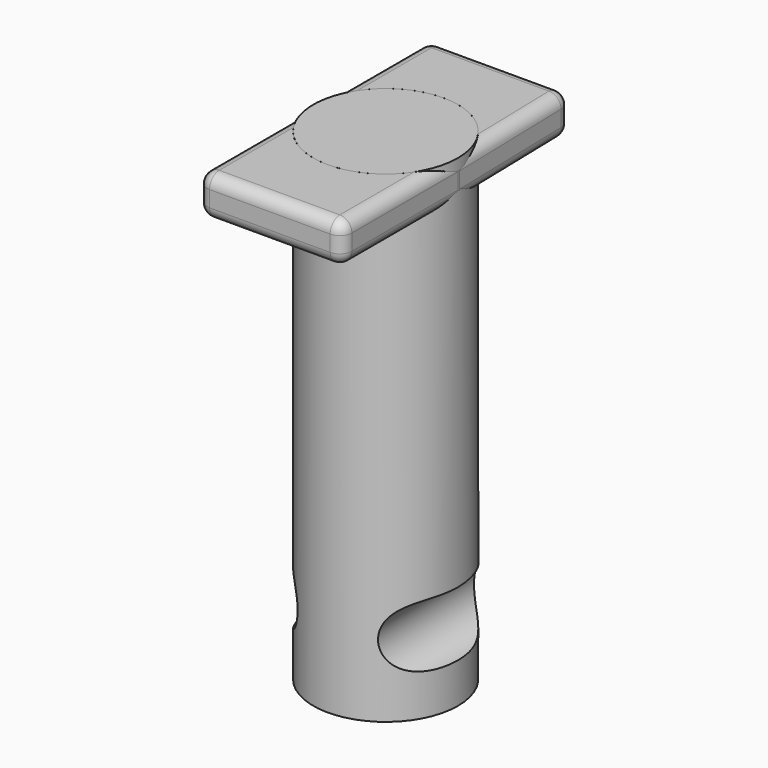
from build123d import *

# Parameters (mm, degrees)
F0_R          = 9
F1_DEPTH      = 60
F2_R          = 4
F3_DEPTH      = 12.55118
F3_DEPTH_BACK = 46.0374
F5_DEPTH      = 5
F6_T1_DEPTH   = 22.875
F6_T3_DEPTH   = 20.25
F6_T5_DEPTH   = 15.002743
F6_T7_DEPTH   = 2
F6_S11_W      = 1.5
F6_S11_H      = 1.5
F6_T12_DEPTH  = 1.5
F6_S17_W      = 1.5
F6_S17_H      = 1.5
F6_T18_DEPTH  = 1.5
F6_S23_W      = 1.5
F6_S23_H      = 1.5
F6_T24_DEPTH  = 1.5
F6_S29_W      = 1.5
F6_S29_H      = 1.5
F6_T30_DEPTH  = 1.5
F6_2_F1_R     = 1.5
F6_2_F2_R     = 1.5
F6_2_F3_R     = 1.5
F6_2_F4_R     = 1.5


# Not quite as in the source:
# - a fillet or chamfer that OpenCascade refuses, or shapes differently, is made with other operations: its cross-section is extruded or revolved along the edge and cut away or added


with BuildPart() as f1:
    # F0 (on Top) → F1 (new body)
    with BuildSketch(Plane.XY):
        Circle(F0_R)
    extrude(amount=F1_DEPTH)

    # F2 (on Front) → F3 (cut, two sides)
    with BuildSketch(Plane.XZ) as f3_sk:
        with Locations((-8.93038, 9)):
            Circle(F2_R)
        with Locations((9.026195, 9)):
            Circle(F2_R)
    extrude(amount=F3_DEPTH, mode=Mode.SUBTRACT)
    extrude(f3_sk.sketch, amount=-F3_DEPTH_BACK, mode=Mode.SUBTRACT)


with BuildPart() as f5:
    # F4 (on face) → F5 (new body)
    with BuildSketch(Plane.XY.offset(60)):
        with BuildLine():
            ThreePointArc((9, 0), (0, -9), (-9, 0))
            Line((-9, 0), (-9, -18))
            Line((-9, -18), (9.002743, -18))
            Line((9.002743, -18), (9.002743, 0))
            Line((9.002743, 0), (8.997257, 0.222169))
            ThreePointArc((8.997257, 0.222169), (8.999314, 0.111093), (9, 0))
        make_face()
    extrude(amount=-F5_DEPTH)

    # F6: fillet of radius 1.5 on 8 edges, made by hand

    # F6_s2 → F6_t1 (cut)
    with BuildSketch(Plane.XZ.offset(-6.375)):
        with BuildLine():
            ThreePointArc((-7.5, 60), (-8.56066, 59.56066), (-9, 58.5))
            Line((-9, 58.5), (-9, 60))
            Line((-9, 60), (-7.5, 60))
        make_face()
        with BuildLine():
            ThreePointArc((-9, 56.5), (-8.56066, 55.43934), (-7.5, 55))
            Line((-7.5, 55), (-9, 55))
            Line((-9, 55), (-9, 56.5))
        make_face()
    extrude(amount=F6_T1_DEPTH, mode=Mode.SUBTRACT)

    # F6_s4 → F6_t3 (cut)
    with BuildSketch(Plane.XZ.offset(-3.75)):
        with BuildLine():
            ThreePointArc((7.502743, 60), (8.563404, 59.56066), (9.002743, 58.5))
            Line((9.002743, 58.5), (9.002743, 60))
            Line((9.002743, 60), (7.502743, 60))
        make_face()
        with BuildLine():
            ThreePointArc((9.002743, 56.5), (8.563404, 55.43934), (7.502743, 55))
            Line((7.502743, 55), (9.002743, 55))
            Line((9.002743, 55), (9.002743, 56.5))
        make_face()
    extrude(amount=F6_T3_DEPTH, mode=Mode.SUBTRACT)

    # F6_s6 → F6_t5 (cut)
    with BuildSketch(Plane.YZ.offset(-7.5)):
        with BuildLine():
            ThreePointArc((-16.5, 60), (-17.56066, 59.56066), (-18, 58.5))
            Line((-18, 58.5), (-18, 60))
            Line((-18, 60), (-16.5, 60))
        make_face()
        with BuildLine():
            ThreePointArc((-18, 56.5), (-17.56066, 55.43934), (-16.5, 55))
            Line((-16.5, 55), (-18, 55))
            Line((-18, 55), (-18, 56.5))
        make_face()
    extrude(amount=F6_T5_DEPTH, mode=Mode.SUBTRACT)

    # F6_s8 → F6_t7 (cut)
    with BuildSketch(Plane.XY.offset(56.5)):
        with BuildLine():
            ThreePointArc((9.002743, -16.5), (8.563404, -17.56066), (7.502743, -18))
            Line((7.502743, -18), (9.002743, -18))
            Line((9.002743, -18), (9.002743, -16.5))
        make_face()
        with BuildLine():
            ThreePointArc((-7.5, -18), (-8.56066, -17.56066), (-9, -16.5))
            Line((-9, -16.5), (-9, -18))
            Line((-9, -18), (-7.5, -18))
        make_face()
    extrude(amount=F6_T7_DEPTH, mode=Mode.SUBTRACT)


with BuildPart() as f5b:
    # F4 (on face) → F5, piece 2 (new body)
    with BuildSketch(Plane.XY.offset(60)):
        with BuildLine():
            Line((-9, 18), (-9, 0))
            ThreePointArc((-9, 0), (-0.111093, 8.999314), (8.997257, 0.222169))
            Line((8.997257, 0.222169), (8.558269, 18))
            Line((8.558269, 18), (-9, 18))
        make_face()
    extrude(amount=-F5_DEPTH)

    # F6#2: fillet of radius 1.5 on 8 edges, made by hand

    # F6_2_f1
    f6_2_f1_edges = [f5b.edges().sort_by_distance(p)[0] for p in [
        (8.558269, 18, 57.5),
    ]]
    fillet(f6_2_f1_edges, radius=F6_2_F1_R)

    # F6_2_f2
    f6_2_f2_edges = [f5b.edges().sort_by_distance(p)[0] for p in [
        (8.795826, 8.379599, 60),
    ]]
    fillet(f6_2_f2_edges, radius=F6_2_F2_R)

    # F6_2_f3
    f6_2_f3_edges = [f5b.edges().sort_by_distance(p)[0] for p in [
        (8.795826, 8.379599, 55),
    ]]
    fillet(f6_2_f3_edges, radius=F6_2_F3_R)

    # F6_2_f4
    f6_2_f4_edges = [f5b.edges().sort_by_distance(p)[0] for p in [
        (-9, 18, 57.5),
    ]]
    fillet(f6_2_f4_edges, radius=F6_2_F4_R)


with BuildPart() as f6_tool10:
    # F6_s11 → F6_t12 (new body)
    with BuildSketch(Plane.XY.offset(58.5)):
        with Locations((-8.25, -17.25)):
            Rectangle(F6_S11_W, F6_S11_H)
    extrude(amount=F6_T12_DEPTH)

    # F6_s13 → F6_t14 (revolve, cut)
    with BuildSketch(Plane(origin=(-7.5, -16.5, 58.5), x_dir=(0.707107, 0.707107, 0), z_dir=(0.707107, -0.707107, 0))):
        with BuildLine():
            ThreePointArc((0, -1.5), (1.5, 0), (0, 1.5))
            Line((0, 1.5), (0, -1.5))
        make_face()
    revolve(axis=Axis((-7.5, -16.5, 58.5), (0, 0, 1)), mode=Mode.SUBTRACT)


with BuildPart() as f5_1:
    add(f5.part)

    # F6_t9: cut F6_tool10
    add(f6_tool10.part, mode=Mode.SUBTRACT)


with BuildPart() as f6_tool16:
    # F6_s17 → F6_t18 (new body)
    with BuildSketch(Plane.XY.offset(58.5)):
        with Locations((8.252743, -17.25)):
            Rectangle(F6_S17_W, F6_S17_H)
    extrude(amount=F6_T18_DEPTH)

    # F6_s19 → F6_t20 (revolve, cut)
    with BuildSketch(Plane(origin=(7.502743, -16.5, 58.5), x_dir=(-0.707107, 0.707107, 0), z_dir=(0.707107, 0.707107, 0))):
        with BuildLine():
            ThreePointArc((0, -1.5), (1.5, 0), (0, 1.5))
            Line((0, 1.5), (0, -1.5))
        make_face()
    revolve(axis=Axis((7.502743, -16.5, 58.5), (0, 0, 1)), mode=Mode.SUBTRACT)


with BuildPart() as f5_2:
    add(f5_1.part)

    # F6_t15: cut F6_tool16
    add(f6_tool16.part, mode=Mode.SUBTRACT)


with BuildPart() as f6_tool22:
    # F6_s23 → F6_t24 (new body)
    with BuildSketch(Plane.XZ.offset(16.5)):
        with Locations((-8.25, 55.75)):
            Rectangle(F6_S23_W, F6_S23_H)
    extrude(amount=F6_T24_DEPTH)

    # F6_s25 → F6_t26 (revolve, cut)
    with BuildSketch(Plane(origin=(-7.5, -16.5, 56.5), x_dir=(0.707107, 0, 0.707107), z_dir=(0.707107, 0, -0.707107))):
        with BuildLine():
            ThreePointArc((0, -1.5), (1.5, 0), (0, 1.5))
            Line((0, 1.5), (0, -1.5))
        make_face()
    revolve(axis=Axis((-7.5, -16.5, 56.5), (0, -1, 0)), mode=Mode.SUBTRACT)


with BuildPart() as f5_3:
    add(f5_2.part)

    # F6_t21: cut F6_tool22
    add(f6_tool22.part, mode=Mode.SUBTRACT)


with BuildPart() as f6_tool28:
    # F6_s29 → F6_t30 (new body)
    with BuildSketch(Plane.YZ.offset(7.502743)):
        with Locations((-17.25, 55.75)):
            Rectangle(F6_S29_W, F6_S29_H)
    extrude(amount=F6_T30_DEPTH)

    # F6_s31 → F6_t32 (revolve, cut)
    with BuildSketch(Plane(origin=(7.502743, -16.5, 56.5), x_dir=(0, 0.707107, 0.707107), z_dir=(0, 0.707107, -0.707107))):
        with BuildLine():
            ThreePointArc((0, -1.5), (1.5, 0), (0, 1.5))
            Line((0, 1.5), (0, -1.5))
        make_face()
    revolve(axis=Axis((7.502743, -16.5, 56.5), (1, 0, 0)), mode=Mode.SUBTRACT)


with BuildPart() as f5_4:
    add(f5_3.part)

    # F6_t27: cut F6_tool28
    add(f6_tool28.part, mode=Mode.SUBTRACT)


solid = Compound([f1.part, f5b.part, f5_4.part])
